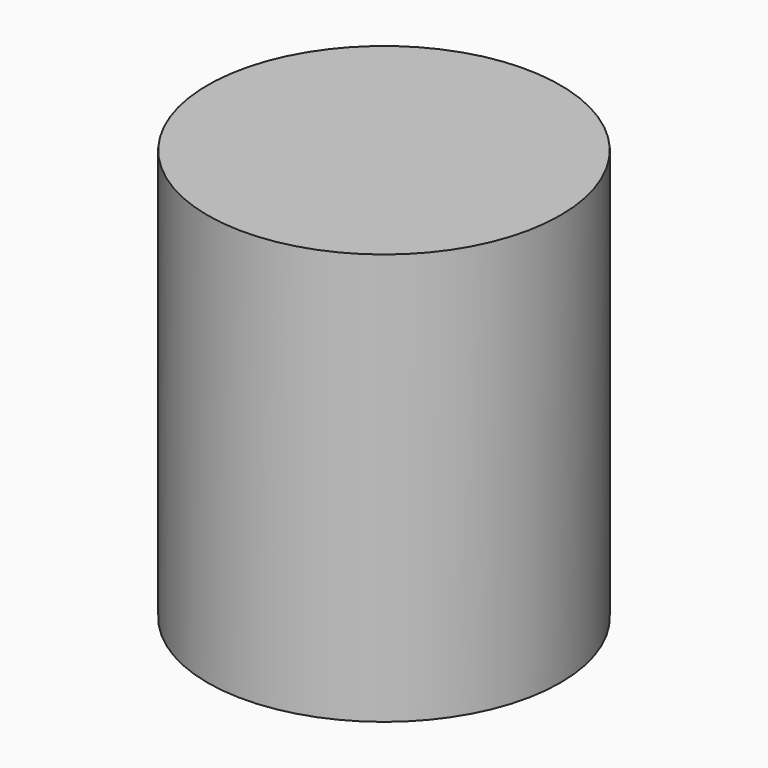
from build123d import *

# Parameters (mm, degrees)
F0_R     = 4.7625
F1_DEPTH = 5.55625


# Not quite as in the source:
# - a length typed as a fraction of an inch, garbled in the dataset ("3 / 203.2 mm" for 3/8 in), is restored


with BuildPart() as f1:
    # F0 (on Top) → F1 (new body, symmetric)
    with BuildSketch(Plane.XY):
        Circle(F0_R)
    extrude(amount=F1_DEPTH, both=True)


solid = f1.part
